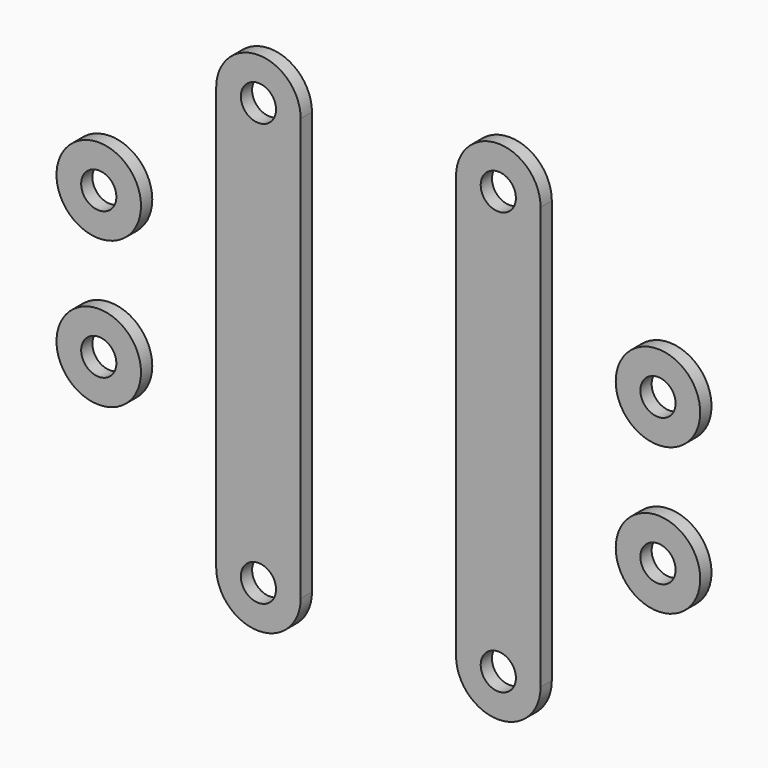
from build123d import *

# Parameters (mm, degrees)
F0_R     = 9.525
F0_R_2   = 3.96875
F1_DEPTH = 3.175
F3_DEPTH = 3.175


with BuildPart() as f1:
    # F0 (on Front) → F1 (new body)
    with BuildSketch(Plane.XZ):
        with Locations((-63.0381852388, 36.9386635721)):
            Circle(F0_R)
        with Locations((-63.0381852388, 36.9386635721)):
            Circle(F0_R_2, mode=Mode.SUBTRACT)
    extrude(amount=F1_DEPTH)


with BuildPart() as f1b:
    # F0 (on Front) → F1, piece 2 (new body)
    with BuildSketch(Plane.XZ):
        with Locations((-63.0381852388, 3.9061459247)):
            Circle(F0_R)
        with Locations((-63.0381852388, 3.9061459247)):
            Circle(F0_R_2, mode=Mode.SUBTRACT)
    extrude(amount=F1_DEPTH)


with BuildPart() as f1c:
    # F0 (on Front) → F1, piece 3 (new body)
    with BuildSketch(Plane.XZ):
        with BuildLine():
            ThreePointArc((-17.5126310602, 65.9878742009), (-27.0376310602, 75.5128742009), (-36.5626310602, 65.9878742009))
            Line((-36.5626310602, 65.9878742009), (-36.5626310602, -29.2621257991))
            ThreePointArc((-36.5626310602, -29.2621257991), (-27.0376310602, -38.7871257991), (-17.5126310602, -29.2621257991))
            Line((-17.5126310602, -29.2621257991), (-17.5126310602, 65.9878742009))
        make_face()
        with Locations((-27.0376310602, -29.2621257991)):
            Circle(F0_R_2, mode=Mode.SUBTRACT)
        with Locations((-27.0376310602, 65.9878742009)):
            Circle(F0_R_2, mode=Mode.SUBTRACT)
    extrude(amount=F1_DEPTH)


with BuildPart() as f2_1:
    # F2: instance of F1c
    add(f1c.part.mirror(Plane.YZ))


with BuildPart() as f3:
    # F0 (on Front) → F3 (new body)
    with BuildSketch(Plane.XZ):
        with Locations((-63.0381852388, 36.9386635721)):
            Circle(F0_R)
        with Locations((-63.0381852388, 36.9386635721)):
            Circle(F0_R_2, mode=Mode.SUBTRACT)
    extrude(amount=F3_DEPTH)


with BuildPart() as f3b:
    # F0 (on Front) → F3, piece 2 (new body)
    with BuildSketch(Plane.XZ):
        with Locations((-63.0381852388, 3.9061459247)):
            Circle(F0_R)
        with Locations((-63.0381852388, 3.9061459247)):
            Circle(F0_R_2, mode=Mode.SUBTRACT)
    extrude(amount=F3_DEPTH)


with BuildPart() as f4_1:
    # F4: instance of F3
    add(f3.part.mirror(Plane.YZ))


with BuildPart() as f4_2:
    # F4: instance of F3b
    add(f3b.part.mirror(Plane.YZ))


solid = Compound([f1.part, f1b.part, f1c.part, f2_1.part, f3.part, f3b.part, f4_1.part, f4_2.part])
